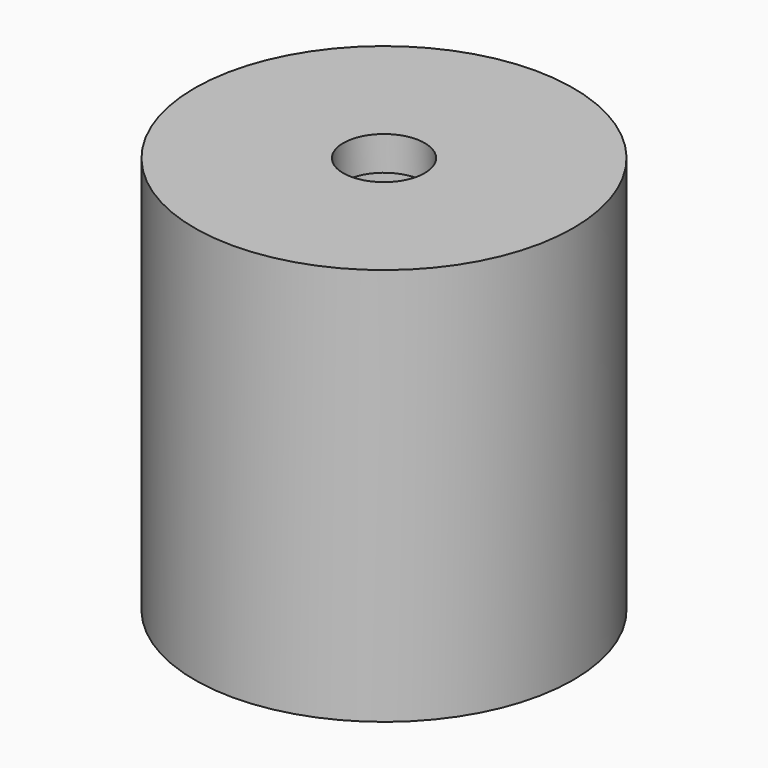
from build123d import *

# Parameters (mm, degrees)
F0_R           = 10
F0_R_2         = 6.3
F1_DEPTH       = 6
F2_DEPTH       = 15
F4_R           = 1
F1_FACE_R      = 10
F7_D           = 4.3
F7_CBORE_D     = 8
F7_CBORE_DEPTH = 4.2
F8_D           = 3.2
F8_DEPTH       = 8
F8_START       = 6
F8_TIP         = 0.9613769904


with BuildPart() as f1:
    # F0 (on Top) → F1 (new body)
    with BuildSketch(Plane.XY):
        Circle(F0_R)
        Circle(F0_R_2, mode=Mode.SUBTRACT)
        Circle(F0_R_2)
    extrude(amount=F1_DEPTH)

    # F0 (on Top) → F2 (join)
    with BuildSketch(Plane.XY):
        Circle(F0_R)
        Circle(F0_R_2, mode=Mode.SUBTRACT)
    extrude(amount=-F2_DEPTH)

    # F7 (through all)
    with Locations(Plane(origin=(0, 0, 0), x_dir=(1, 0, 0), z_dir=(0, 0, -1))):
        with Locations((0, 0)):
            CounterBoreHole(F7_D / 2, F7_CBORE_D / 2, F7_CBORE_DEPTH)


with BuildPart() as f5:
    # F4 (on offset) → F5 section 0
    with BuildSketch(Plane.XY.offset(16)):
        Circle(F4_R)
    # F1_face (on face) → F5 section 1
    with BuildSketch(Plane.XY.offset(6)):
        Circle(F1_FACE_R)
    loft()

    # F8
    # its depths count from where the whole tool has entered the part; down to there all is cleared
    with Locations(Plane(origin=(0, 0, 0), x_dir=(1, 0, 0), z_dir=(0, 0, -1)).offset(-F8_START)):
        with Locations((0, 0)):
            Hole(F8_D / 2, depth=F8_DEPTH)
            with Locations((0, 0, -(F8_DEPTH + F8_TIP / 2))):  # 118° drill point
                Cone(0, F8_D / 2, F8_TIP, mode=Mode.SUBTRACT)


solid = f1.part
